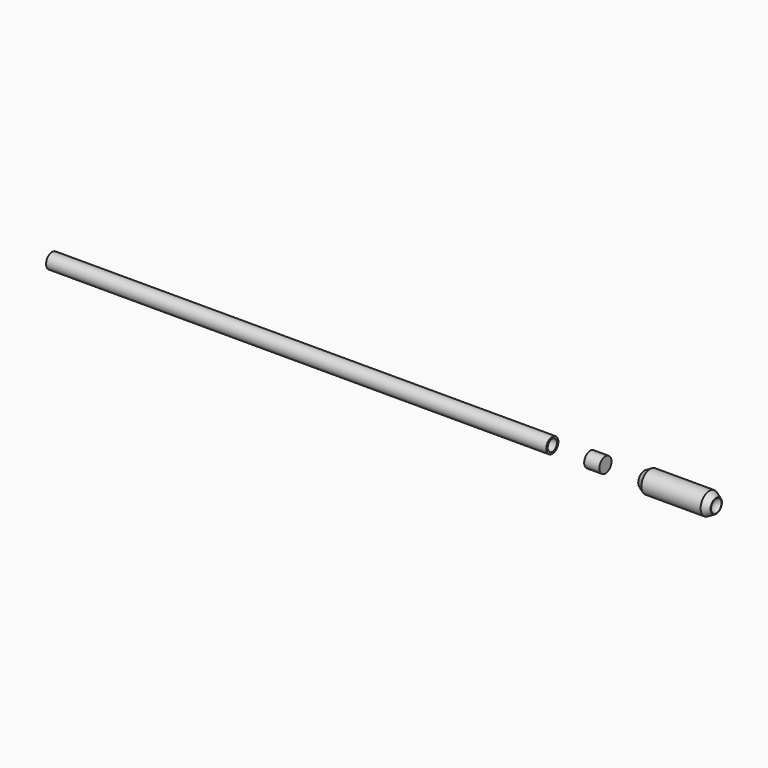
from build123d import *

# Parameters (mm, degrees)
F3_R     = 5
F4_DEPTH = 10
F6_R     = 5
F6_R_2   = 3.8
F7_DEPTH = 329.475


# Not quite as in the source:
# - a fillet or chamfer that OpenCascade refuses, or shapes differently, is made with other operations: its cross-section is extruded or revolved along the edge and cut away or added


with BuildPart() as f1:
    # F0 (on Front) → F1 (revolve)
    with BuildSketch(Plane.XZ):
        with BuildLine():
            Line((-50, -7.2625), (-2, -7.2625))
            Line((-2, -7.2625), (-2, -4.3221992377))
            ThreePointArc((-2, -4.3221992377), (-4.0128796549, -2.5648007964), (-4.7625, 0))
            Line((-4.7625, 0), (-5.2625, 0))
            Line((-5.2625, 0), (-5.2625, -5))
            Line((-5.2625, -5), (-50, -5))
            Line((-50, -5), (-50, -7.2625))
        make_face()
    revolve(axis=Axis((-5.0125, 0, 0), (-1, 0, 0)))

    # F8: chamfer of 4.5 x 2.5980762114 on 2 edges, made by hand

    # F8_s1 → F8_t2 (revolve, cut)
    with BuildSketch(Plane.XZ):
        Polygon((-50, -4.6644237886), (-45.5, -7.2625), (-50, -7.2625), align=None)
    revolve(axis=Axis((-50, 0, 0), (-1, 0, 0)), mode=Mode.SUBTRACT)

    # F8_s3 → F8_t4 (revolve, cut)
    with BuildSketch(Plane.XZ):
        Polygon((-6.5, -7.2625), (-2, -4.6644237886), (-2, -7.2625), align=None)
    revolve(axis=Axis((-2, 0, 0), (-1, 0, 0)), mode=Mode.SUBTRACT)


with BuildPart() as f4:
    # F3 (on offset) → F4 (new body)
    with BuildSketch(Plane(origin=(-75, 0, 0), x_dir=(0, -1, 0), z_dir=(-1, 0, 0))):
        Circle(F3_R)
    extrude(amount=F4_DEPTH)


with BuildPart() as f7:
    # F6 (on offset) → F7 (new body)
    with BuildSketch(Plane(origin=(-110, 0, 0), x_dir=(0, -1, 0), z_dir=(-1, 0, 0))):
        Circle(F6_R)
        Circle(F6_R_2, mode=Mode.SUBTRACT)
    extrude(amount=F7_DEPTH)


solid = Compound([f1.part, f4.part, f7.part])
